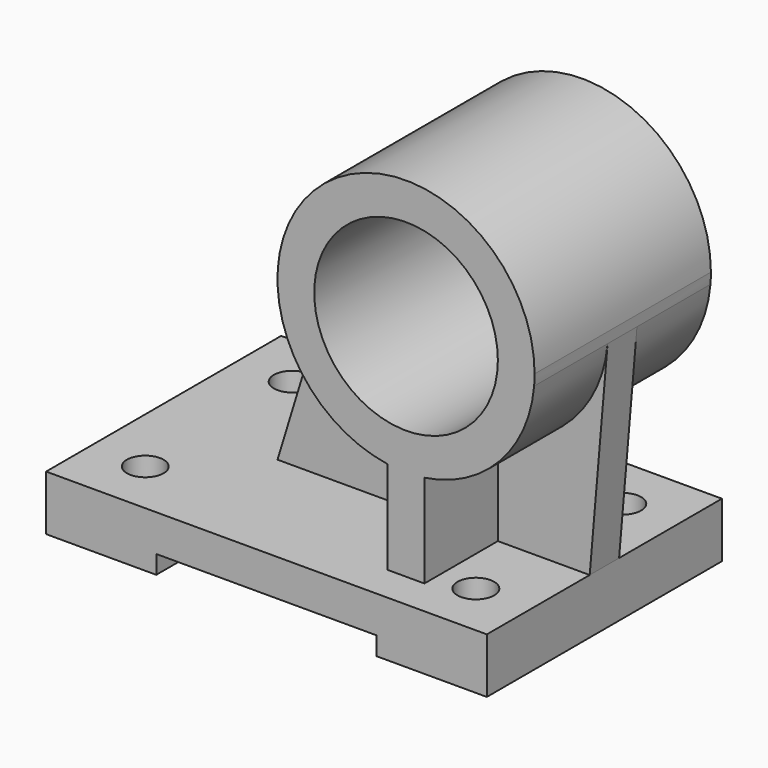
from build123d import *
from build123d import SkipClean  # not in build123d's __all__

# Parameters (mm, degrees)
F0_R      = 25
F1_DEPTH  = 40
F2_R      = 25
F3_DEPTH  = 10
F4_R      = 25
F5_DEPTH  = 10
F7_DEPTH  = 25
F9_DEPTH  = 25
F11_D     = 10
F11_DEPTH = 16.5
F11_TIP   = 3.0043030951


with BuildPart() as f1:
    # F0 (on Front) → F1 (new body, symmetric)
    with BuildSketch(Plane.XZ):
        Polygon((0, 15), (0, 0), (30, 0), (30, 5), (90, 5), (90, 0), (120, 0), (120, 15), (35, 15), align=None)
        with BuildLine():
            Line((56.536927729, 85.2578162484), (35, 15))
            Line((35, 15), (120, 15))
            Line((120, 15), (124.8728873319, 72.0197769993))
            ThreePointArc((124.8728873319, 72.0197769993), (83.3435508402, 40.638805542), (56.536927729, 85.2578162484))
        make_face()
        with BuildLine():
            ThreePointArc((125, 75), (95.186158044, 109.613635532), (56.536927729, 85.2578162484))
            ThreePointArc((56.536927729, 85.2578162484), (83.3435508402, 40.638805542), (124.8728873319, 72.0197769993))
            ThreePointArc((124.8728873319, 72.0197769993), (124.9682073934, 73.5085337111), (125, 75))
        make_face()
        with Locations((90, 75)):
            Circle(F0_R, mode=Mode.SUBTRACT)
    extrude(amount=F1_DEPTH, both=True)

    # F2 (on face) → F3 (cut)
    with BuildSketch(Plane.XZ.offset(40)):
        with BuildLine():
            Line((56.536927729, 85.2578162484), (35, 15))
            Line((35, 15), (120, 15))
            Line((120, 15), (124.8728873319, 72.0197769993))
            ThreePointArc((124.8728873319, 72.0197769993), (96.6564491598, 109.361194458), (56.536927729, 85.2578162484))
        make_face()
        with Locations((90, 75)):
            Circle(F2_R, mode=Mode.SUBTRACT)
    extrude(amount=-F3_DEPTH, mode=Mode.SUBTRACT)

    # F4 (on face) → F5 (cut)
    with BuildSketch(Plane(origin=(0, 40, 0), x_dir=(-1, 0, 0), z_dir=(0, 1, 0))):
        with BuildLine():
            Line((-120, 15), (-35, 15))
            Line((-35, 15), (-56.536927729, 85.2578162484))
            ThreePointArc((-56.536927729, 85.2578162484), (-96.6564491598, 109.361194458), (-124.8728873319, 72.0197769993))
            Line((-124.8728873319, 72.0197769993), (-120, 15))
        make_face()
        with Locations((-90, 75)):
            Circle(F4_R, mode=Mode.SUBTRACT)
    extrude(amount=-F5_DEPTH, mode=Mode.SUBTRACT)

    # F6 (on face) → F7 (cut)
    with BuildSketch(Plane.XZ.offset(30)):
        with BuildLine():
            ThreePointArc((85, 40.3589838486), (60.439413574, 56.2604234265), (56.536927729, 85.2578162484))
            Line((56.536927729, 85.2578162484), (35, 15))
            Line((35, 15), (85, 15))
            Line((85, 15), (85, 40.3589838486))
        make_face()
        with BuildLine():
            Line((120, 15), (124.8728873319, 72.0197769993))
            ThreePointArc((124.8728873319, 72.0197769993), (115.4570862783, 50.980492132), (95, 40.3589838486))
            Line((95, 40.3589838486), (95, 15))
            Line((95, 15), (120, 15))
        make_face()
    with SkipClean():  # cleaning this boolean's faces spoils the solid; the shape is the same uncleaned
        extrude(amount=-F7_DEPTH, mode=Mode.SUBTRACT)

    # F8 (on face) → F9 (cut)
    with BuildSketch(Plane(origin=(0, 30, 0), x_dir=(-1, 0, 0), z_dir=(0, 1, 0))):
        with BuildLine():
            ThreePointArc((-95, 40.3589838486), (-115.4570862783, 50.980492132), (-124.8728873319, 72.0197769993))
            Line((-124.8728873319, 72.0197769993), (-120, 15))
            Line((-120, 15), (-95, 15))
            Line((-95, 15), (-95, 40.3589838486))
        make_face()
        with BuildLine():
            Line((-35, 15), (-56.536927729, 85.2578162484))
            ThreePointArc((-56.536927729, 85.2578162484), (-60.439413574, 56.2604234265), (-85, 40.3589838486))
            Line((-85, 40.3589838486), (-85, 15))
            Line((-85, 15), (-35, 15))
        make_face()
    extrude(amount=-F9_DEPTH, mode=Mode.SUBTRACT)

    # F11
    with Locations(Plane.XY.offset(15)):
        with Locations((15, 25), (15, -25), (105, -25), (105, 25)):
            Hole(F11_D / 2, depth=F11_DEPTH)
            with Locations((0, 0, -(F11_DEPTH + F11_TIP / 2))):  # 118° drill point
                Cone(0, F11_D / 2, F11_TIP, mode=Mode.SUBTRACT)


solid = f1.part
